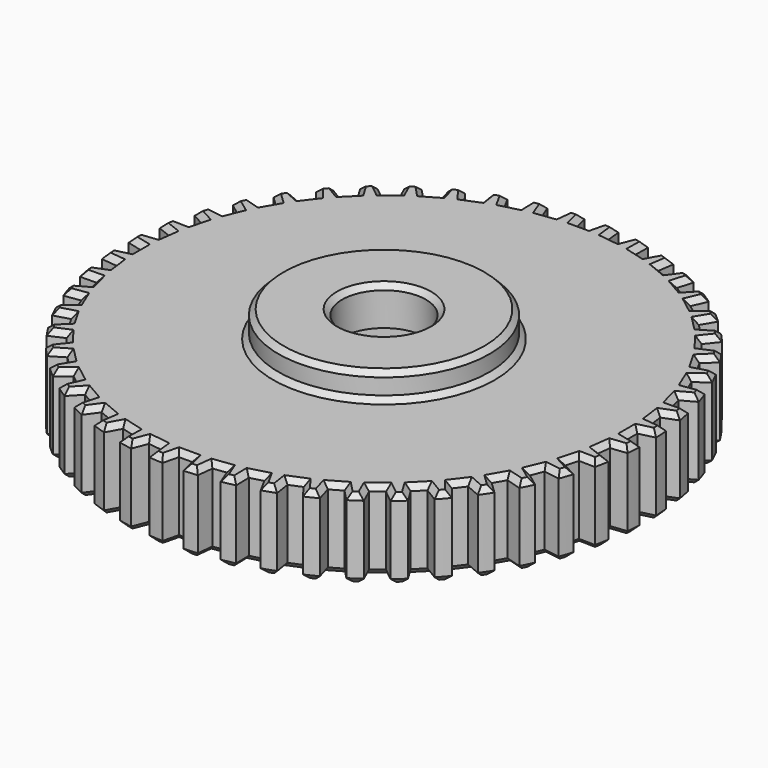
from build123d import *

# Parameters (mm, degrees)
F0_R            = 10
F1_DEPTH        = 3
F2_R            = 4
F3_DEPTH        = 1
F5_DEPTH        = 2.54
F7_DEPTH        = 3.001
F7_COPIES_COUNT = 48
F8_R            = 1.5875
F9_DEPTH        = 4.001
F10_SIZE        = 0.2


# Not quite as in the source:
# - a pattern or mirror of a feature is missing from the dataset's text; its kind, count and spacing are read off the source's solid


with BuildPart() as f1:
    # F0 (on Top) → F1 (new body)
    with BuildSketch(Plane.XY):
        Circle(F0_R)
    extrude(amount=F1_DEPTH)

    # F2 (on face) → F3 (join)
    with BuildSketch(Plane.XY.offset(3)):
        Circle(F2_R)
    extrude(amount=F3_DEPTH)

    # F4 (on face) → F5 (cut)
    with BuildSketch(Plane(origin=(0, 0, 0), x_dir=(1, 0, 0), z_dir=(0, 0, -1))):
        Polygon((-3.0645261044, -1.2230105296), (-0.4731048645, -3.2654627218), (2.5914212399, -2.0424521922), (3.0645261044, 1.2230105296), (0.4731048645, 3.2654627218), (-2.5914212399, 2.0424521922), align=None)
    extrude(amount=-F5_DEPTH, mode=Mode.SUBTRACT)

    # F6 (on face) → F7 (cut, through all)
    with BuildSketch(Plane.XY.offset(3)):
        Polygon((0.5, 10.414), (-0.5, 10.414), (-0.25, 9.398), (0.25, 9.398), align=None)
    f7 = extrude(amount=-F7_DEPTH, mode=Mode.SUBTRACT)

    # F7_copies: F7 ×48 about axis
    f7_copies_axis = Axis((0, 0, 0), (0, 0, 1))
    for i in range(1, F7_COPIES_COUNT):
        add(f7.rotate(f7_copies_axis, i * 360 / F7_COPIES_COUNT), mode=Mode.SUBTRACT)

    # F8 (on face) → F9 (cut, through all)
    with BuildSketch(Plane.XY.offset(4)):
        Circle(F8_R)
    extrude(amount=-F9_DEPTH, mode=Mode.SUBTRACT)

    # F10
    f10_edges = [f1.edges().sort_by_distance(p)[0] for p in [
        (-0.323099, 9.695074, 0),
        (0, 9.398, 0),
        (0.323099, 9.695074, 0),
        (0.654031, 9.978589, 0),
        (0.945126, 9.654304, 0),
        (1.226685, 9.317599, 0),
        (1.585796, 9.569959, 0),
        (1.950903, 9.807853, 0),
        (2.19718, 9.448347, 0),
        (2.432381, 9.077771, 0),
        (2.821359, 9.281098, 0),
        (3.214395, 9.469301, 0),
        (3.41164, 9.080725, 0),
        (3.596459, 8.68262, 0),
        (4.008649, 8.833436, 0),
        (4.422887, 8.968727, 0),
        (4.567725, 8.55773, 0),
        (4.699, 8.138907, 0),
        (5.127349, 8.234631, 0),
        (5.555702, 8.314696, 0),
        (5.645656, 7.88831, 0),
        (5.72114, 7.455935, 0),
        (6.158319, 7.494929, 0),
        (6.593458, 7.518398, 0),
        (6.626987, 7.083918, 0),
        (6.64539, 6.64539, 0),
        (7.083918, 6.626987, 0),
        (7.518398, 6.593458, 0),
        (7.494929, 6.158319, 0),
        (7.455935, 5.72114, 0),
        (7.88831, 5.645656, 0),
        (8.314696, 5.555702, 0),
        (8.234631, 5.127349, 0),
        (8.138907, 4.699, 0),
        (8.55773, 4.567725, 0),
        (8.968727, 4.422887, 0),
        (8.833436, 4.008649, 0),
        (8.68262, 3.596459, 0),
        (9.080725, 3.41164, 0),
        (9.469301, 3.214395, 0),
        (9.281098, 2.821359, 0),
        (9.077771, 2.432381, 0),
        (9.448347, 2.19718, 0),
        (9.807853, 1.950903, 0),
        (9.569959, 1.585796, 0),
        (9.317599, 1.226685, 0),
        (9.654304, 0.945126, 0),
        (9.978589, 0.654031, 0),
        (9.695074, 0.323099, 0),
        (9.398, 0, 0),
        (9.695074, -0.323099, 0),
        (9.978589, -0.654031, 0),
        (9.654304, -0.945126, 0),
        (9.317599, -1.226685, 0),
        (9.569959, -1.585796, 0),
        (9.807853, -1.950903, 0),
        (9.448347, -2.19718, 0),
        (9.077771, -2.432381, 0),
        (9.281098, -2.821359, 0),
        (9.469301, -3.214395, 0),
        (9.080725, -3.41164, 0),
        (8.68262, -3.596459, 0),
        (8.833436, -4.008649, 0),
        (8.968727, -4.422887, 0),
        (8.55773, -4.567725, 0),
        (8.138907, -4.699, 0),
        (8.234631, -5.127349, 0),
        (8.314696, -5.555702, 0),
        (7.88831, -5.645656, 0),
        (7.455935, -5.72114, 0),
        (7.494929, -6.158319, 0),
        (7.518398, -6.593458, 0),
        (7.083918, -6.626987, 0),
        (6.64539, -6.64539, 0),
        (6.626987, -7.083918, 0),
        (6.593458, -7.518398, 0),
        (6.158319, -7.494929, 0),
        (5.72114, -7.455935, 0),
        (5.645656, -7.88831, 0),
        (5.555702, -8.314696, 0),
        (5.127349, -8.234631, 0),
        (4.699, -8.138907, 0),
        (4.567725, -8.55773, 0),
        (4.422887, -8.968727, 0),
        (4.008649, -8.833436, 0),
        (3.596459, -8.68262, 0),
        (3.41164, -9.080725, 0),
        (3.214395, -9.469301, 0),
        (2.821359, -9.281098, 0),
        (2.432381, -9.077771, 0),
        (2.19718, -9.448347, 0),
        (1.950903, -9.807853, 0),
        (1.585796, -9.569959, 0),
        (1.226685, -9.317599, 0),
        (0.945126, -9.654304, 0),
        (0.654031, -9.978589, 0),
        (0.323099, -9.695074, 0),
        (0, -9.398, 0),
        (-0.323099, -9.695074, 0),
        (-0.654031, -9.978589, 0),
        (-0.945126, -9.654304, 0),
        (-1.226685, -9.317599, 0),
        (-1.585796, -9.569959, 0),
        (-1.950903, -9.807853, 0),
        (-2.19718, -9.448347, 0),
        (-2.432381, -9.077771, 0),
        (-2.821359, -9.281098, 0),
        (-3.214395, -9.469301, 0),
        (-3.41164, -9.080725, 0),
        (-3.596459, -8.68262, 0),
        (-4.008649, -8.833436, 0),
        (-4.422887, -8.968727, 0),
        (-4.567725, -8.55773, 0),
        (-4.699, -8.138907, 0),
        (-5.127349, -8.234631, 0),
        (-5.555702, -8.314696, 0),
        (-5.645656, -7.88831, 0),
        (-5.72114, -7.455935, 0),
        (-6.158319, -7.494929, 0),
        (-6.593458, -7.518398, 0),
        (-6.626987, -7.083918, 0),
        (-6.64539, -6.64539, 0),
        (-7.083918, -6.626987, 0),
        (-7.518398, -6.593458, 0),
        (-7.494929, -6.158319, 0),
        (-7.455935, -5.72114, 0),
        (-7.88831, -5.645656, 0),
        (-8.314696, -5.555702, 0),
        (-8.234631, -5.127349, 0),
        (-8.138907, -4.699, 0),
        (-8.55773, -4.567725, 0),
        (-8.968727, -4.422887, 0),
        (-8.833436, -4.008649, 0),
        (-8.68262, -3.596459, 0),
        (-9.080725, -3.41164, 0),
        (-9.469301, -3.214395, 0),
        (-9.281098, -2.821359, 0),
        (-9.077771, -2.432381, 0),
        (-9.448347, -2.19718, 0),
        (-9.807853, -1.950903, 0),
        (-9.569959, -1.585796, 0),
        (-9.317599, -1.226685, 0),
        (-9.654304, -0.945126, 0),
        (-9.978589, -0.654031, 0),
        (-9.695074, -0.323099, 0),
        (-9.398, 0, 0),
        (-9.695074, 0.323099, 0),
        (-9.978589, 0.654031, 0),
        (-9.654304, 0.945126, 0),
        (-9.317599, 1.226685, 0),
        (-9.569959, 1.585796, 0),
        (-9.807853, 1.950903, 0),
        (-9.448347, 2.19718, 0),
        (-9.077771, 2.432381, 0),
        (-9.281098, 2.821359, 0),
        (-9.469301, 3.214395, 0),
        (-9.080725, 3.41164, 0),
        (-8.68262, 3.596459, 0),
        (-8.833436, 4.008649, 0),
        (-8.968727, 4.422887, 0),
        (-8.55773, 4.567725, 0),
        (-8.138907, 4.699, 0),
        (-8.234631, 5.127349, 0),
        (-8.314696, 5.555702, 0),
        (-7.88831, 5.645656, 0),
        (-7.455935, 5.72114, 0),
        (-7.494929, 6.158319, 0),
        (-7.518398, 6.593458, 0),
        (-7.083918, 6.626987, 0),
        (-6.64539, 6.64539, 0),
        (-6.626987, 7.083918, 0),
        (-6.593458, 7.518398, 0),
        (-6.158319, 7.494929, 0),
        (-5.72114, 7.455935, 0),
        (-5.645656, 7.88831, 0),
        (-5.555702, 8.314696, 0),
        (-5.127349, 8.234631, 0),
        (-4.699, 8.138907, 0),
        (-4.567725, 8.55773, 0),
        (-4.422887, 8.968727, 0),
        (-4.008649, 8.833436, 0),
        (-3.596459, 8.68262, 0),
        (-3.41164, 9.080725, 0),
        (-3.214395, 9.469301, 0),
        (-2.821359, 9.281098, 0),
        (-2.432381, 9.077771, 0),
        (-2.19718, 9.448347, 0),
        (-1.950903, 9.807853, 0),
        (-1.585796, 9.569959, 0),
        (-1.226685, 9.317599, 0),
        (-0.945126, 9.654304, 0),
        (-0.654031, 9.978589, 0),
        (-2.827974, -0.409721, 0),
        (-1.059158, -2.653957, 0),
        (-1.768815, 2.244237, 0),
        (1.768815, -2.244237, 0),
        (1.059158, 2.653957, 0),
        (2.827974, 0.409721, 0),
        (-0.323099, 9.695074, 3),
        (0, 9.398, 3),
        (0.323099, 9.695074, 3),
        (0.654031, 9.978589, 3),
        (0.945126, 9.654304, 3),
        (1.226685, 9.317599, 3),
        (1.585796, 9.569959, 3),
        (1.950903, 9.807853, 3),
        (2.19718, 9.448347, 3),
        (2.432381, 9.077771, 3),
        (2.821359, 9.281098, 3),
        (3.214395, 9.469301, 3),
        (3.41164, 9.080725, 3),
        (3.596459, 8.68262, 3),
        (4.008649, 8.833436, 3),
        (4.422887, 8.968727, 3),
        (4.567725, 8.55773, 3),
        (4.699, 8.138907, 3),
        (5.127349, 8.234631, 3),
        (5.555702, 8.314696, 3),
        (5.645656, 7.88831, 3),
        (5.72114, 7.455935, 3),
        (6.158319, 7.494929, 3),
        (6.593458, 7.518398, 3),
        (6.626987, 7.083918, 3),
        (6.64539, 6.64539, 3),
        (7.083918, 6.626987, 3),
        (7.518398, 6.593458, 3),
        (7.494929, 6.158319, 3),
        (7.455935, 5.72114, 3),
        (7.88831, 5.645656, 3),
        (8.314696, 5.555702, 3),
        (8.234631, 5.127349, 3),
        (8.138907, 4.699, 3),
        (8.55773, 4.567725, 3),
        (8.968727, 4.422887, 3),
        (8.833436, 4.008649, 3),
        (8.68262, 3.596459, 3),
        (9.080725, 3.41164, 3),
        (9.469301, 3.214395, 3),
        (9.281098, 2.821359, 3),
        (9.077771, 2.432381, 3),
        (9.448347, 2.19718, 3),
        (9.807853, 1.950903, 3),
        (9.569959, 1.585796, 3),
        (9.317599, 1.226685, 3),
        (9.654304, 0.945126, 3),
        (9.978589, 0.654031, 3),
        (9.695074, 0.323099, 3),
        (9.398, 0, 3),
        (9.695074, -0.323099, 3),
        (9.978589, -0.654031, 3),
        (9.654304, -0.945126, 3),
        (9.317599, -1.226685, 3),
        (9.569959, -1.585796, 3),
        (9.807853, -1.950903, 3),
        (9.448347, -2.19718, 3),
        (9.077771, -2.432381, 3),
        (9.281098, -2.821359, 3),
        (9.469301, -3.214395, 3),
        (9.080725, -3.41164, 3),
        (8.68262, -3.596459, 3),
        (8.833436, -4.008649, 3),
        (8.968727, -4.422887, 3),
        (8.55773, -4.567725, 3),
        (8.138907, -4.699, 3),
        (8.234631, -5.127349, 3),
        (8.314696, -5.555702, 3),
        (7.88831, -5.645656, 3),
        (7.455935, -5.72114, 3),
        (7.494929, -6.158319, 3),
        (7.518398, -6.593458, 3),
        (7.083918, -6.626987, 3),
        (6.64539, -6.64539, 3),
        (6.626987, -7.083918, 3),
        (6.593458, -7.518398, 3),
        (6.158319, -7.494929, 3),
        (5.72114, -7.455935, 3),
        (5.645656, -7.88831, 3),
        (5.555702, -8.314696, 3),
        (5.127349, -8.234631, 3),
        (4.699, -8.138907, 3),
        (4.567725, -8.55773, 3),
        (4.422887, -8.968727, 3),
        (4.008649, -8.833436, 3),
        (3.596459, -8.68262, 3),
        (3.41164, -9.080725, 3),
        (3.214395, -9.469301, 3),
        (2.821359, -9.281098, 3),
        (2.432381, -9.077771, 3),
        (2.19718, -9.448347, 3),
        (1.950903, -9.807853, 3),
        (1.585796, -9.569959, 3),
        (1.226685, -9.317599, 3),
        (0.945126, -9.654304, 3),
        (0.654031, -9.978589, 3),
        (0.323099, -9.695074, 3),
        (0, -9.398, 3),
        (-0.323099, -9.695074, 3),
        (-0.654031, -9.978589, 3),
        (-0.945126, -9.654304, 3),
        (-1.226685, -9.317599, 3),
        (-1.585796, -9.569959, 3),
        (-1.950903, -9.807853, 3),
        (-2.19718, -9.448347, 3),
        (-2.432381, -9.077771, 3),
        (-2.821359, -9.281098, 3),
        (-3.214395, -9.469301, 3),
        (-3.41164, -9.080725, 3),
        (-3.596459, -8.68262, 3),
        (-4.008649, -8.833436, 3),
        (-4.422887, -8.968727, 3),
        (-4.567725, -8.55773, 3),
        (-4.699, -8.138907, 3),
        (-5.127349, -8.234631, 3),
        (-5.555702, -8.314696, 3),
        (-5.645656, -7.88831, 3),
        (-5.72114, -7.455935, 3),
        (-6.158319, -7.494929, 3),
        (-6.593458, -7.518398, 3),
        (-6.626987, -7.083918, 3),
        (-6.64539, -6.64539, 3),
        (-7.083918, -6.626987, 3),
        (-7.518398, -6.593458, 3),
        (-7.494929, -6.158319, 3),
        (-7.455935, -5.72114, 3),
        (-7.88831, -5.645656, 3),
        (-8.314696, -5.555702, 3),
        (-8.234631, -5.127349, 3),
        (-8.138907, -4.699, 3),
        (-8.55773, -4.567725, 3),
        (-8.968727, -4.422887, 3),
        (-8.833436, -4.008649, 3),
        (-8.68262, -3.596459, 3),
        (-9.080725, -3.41164, 3),
        (-9.469301, -3.214395, 3),
        (-9.281098, -2.821359, 3),
        (-9.077771, -2.432381, 3),
        (-9.448347, -2.19718, 3),
        (-9.807853, -1.950903, 3),
        (-9.569959, -1.585796, 3),
        (-9.317599, -1.226685, 3),
        (-9.654304, -0.945126, 3),
        (-9.978589, -0.654031, 3),
        (-9.695074, -0.323099, 3),
        (-9.398, 0, 3),
        (-9.695074, 0.323099, 3),
        (-9.978589, 0.654031, 3),
        (-9.654304, 0.945126, 3),
        (-9.317599, 1.226685, 3),
        (-9.569959, 1.585796, 3),
        (-9.807853, 1.950903, 3),
        (-9.448347, 2.19718, 3),
        (-9.077771, 2.432381, 3),
        (-9.281098, 2.821359, 3),
        (-9.469301, 3.214395, 3),
        (-9.080725, 3.41164, 3),
        (-8.68262, 3.596459, 3),
        (-8.833436, 4.008649, 3),
        (-8.968727, 4.422887, 3),
        (-8.55773, 4.567725, 3),
        (-8.138907, 4.699, 3),
        (-8.234631, 5.127349, 3),
        (-8.314696, 5.555702, 3),
        (-7.88831, 5.645656, 3),
        (-7.455935, 5.72114, 3),
        (-7.494929, 6.158319, 3),
        (-7.518398, 6.593458, 3),
        (-7.083918, 6.626987, 3),
        (-6.64539, 6.64539, 3),
        (-6.626987, 7.083918, 3),
        (-6.593458, 7.518398, 3),
        (-6.158319, 7.494929, 3),
        (-5.72114, 7.455935, 3),
        (-5.645656, 7.88831, 3),
        (-5.555702, 8.314696, 3),
        (-5.127349, 8.234631, 3),
        (-4.699, 8.138907, 3),
        (-4.567725, 8.55773, 3),
        (-4.422887, 8.968727, 3),
        (-4.008649, 8.833436, 3),
        (-3.596459, 8.68262, 3),
        (-3.41164, 9.080725, 3),
        (-3.214395, 9.469301, 3),
        (-2.821359, 9.281098, 3),
        (-2.432381, 9.077771, 3),
        (-2.19718, 9.448347, 3),
        (-1.950903, 9.807853, 3),
        (-1.585796, 9.569959, 3),
        (-1.226685, 9.317599, 3),
        (-0.945126, 9.654304, 3),
        (-0.654031, 9.978589, 3),
        (-4, 0, 3),
        (-4, 0, 4),
        (-1.5875, 0, 4),
    ]]
    chamfer(f10_edges, length=F10_SIZE)


solid = f1.part
